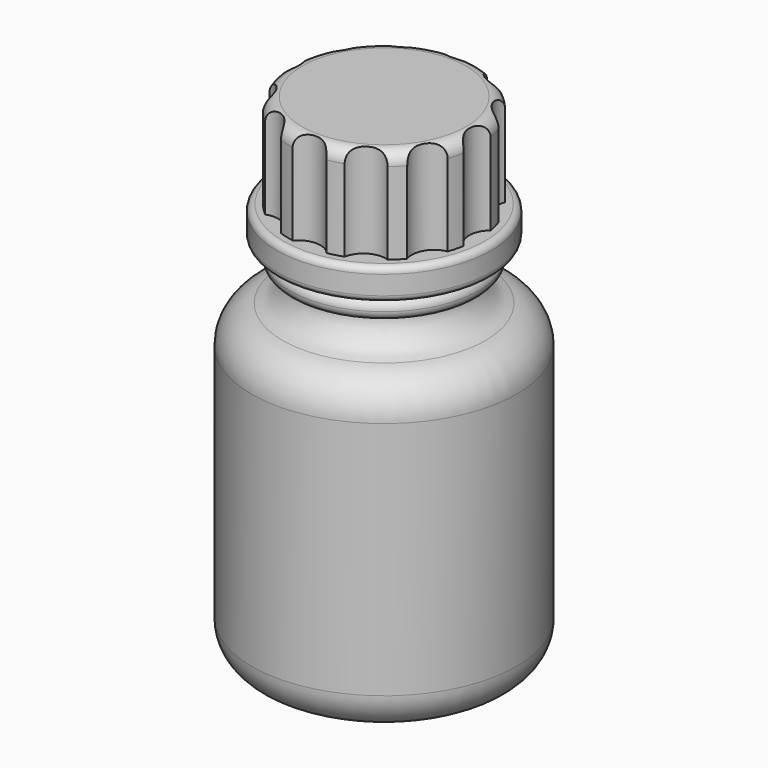
from build123d import *

# Parameters (mm, degrees)
F2_R     = 6
F3_R     = 6
F4_R     = 4.99999
F5_R     = 1.49999
F6_R     = 1
F7_R     = 2
F8_R     = 3.5
F9_DEPTH = 15


# Not quite as in the source:
# - a fillet or chamfer is up to 0.001 mm smaller than in the source, because OpenCascade refuses the exact size


with BuildPart() as f1:
    # F0 (on Front) → F1 (revolve)
    with BuildSketch(Plane.XZ):
        Polygon((-21, 0), (0, 0), (0, 78.75), (-15, 78.75), (-15, 63.75), (-17, 63.75), (-17, 58.75), (-12, 58.75), (-12, 58), (-15, 58), (-15, 55), (-12, 55), (-12, 50), (-21, 50), align=None)
    revolve(axis=Axis((0, 0, 32.9393539578), (0, 0, -1)))

    # F2
    f2_edges = [f1.edges().sort_by_distance(p)[0] for p in [
        (21, 0, 0),
    ]]
    fillet(f2_edges, radius=F2_R)

    # F3
    f3_edges = [f1.edges().sort_by_distance(p)[0] for p in [
        (21, 0, 50),
    ]]
    fillet(f3_edges, radius=F3_R)

    # F4 (radius 5 in the source; OpenCascade refuses exactly that, so slightly less here)
    f4_edges = [f1.edges().sort_by_distance(p)[0] for p in [
        (12, 0, 50),
    ]]
    fillet(f4_edges, radius=F4_R)

    # F5 (radius 1.5 in the source; OpenCascade refuses exactly that, so slightly less here)
    f5_edges = [f1.edges().sort_by_distance(p)[0] for p in [
        (15, 0, 55),
        (15, 0, 58),
    ]]
    fillet(f5_edges, radius=F5_R)

    # F6
    f6_edges = [f1.edges().sort_by_distance(p)[0] for p in [
        (17, 0, 58.75),
        (17, 0, 63.75),
    ]]
    fillet(f6_edges, radius=F6_R)

    # F7
    f7_edges = [f1.edges().sort_by_distance(p)[0] for p in [
        (15, 0, 78.75),
    ]]
    fillet(f7_edges, radius=F7_R)

    # F8 (on face) → F9 (cut)
    with BuildSketch(Plane.XY.offset(78.75)):
        with Locations((0, 17)):
            Circle(F8_R)
        with Locations((-8.5, 14.7224318643)):
            Circle(F8_R)
        with Locations((-14.7224318643, 8.5)):
            Circle(F8_R)
        with Locations((-17, 0)):
            Circle(F8_R)
        with Locations((-14.7224318643, -8.5)):
            Circle(F8_R)
        with Locations((-8.5, -14.7224318643)):
            Circle(F8_R)
        with Locations((0, -17)):
            Circle(F8_R)
        with Locations((8.5, -14.7224318643)):
            Circle(F8_R)
        with Locations((14.7224318643, -8.5)):
            Circle(F8_R)
        with Locations((17, 0)):
            Circle(F8_R)
        with Locations((14.7224318643, 8.5)):
            Circle(F8_R)
        with Locations((8.5, 14.7224318643)):
            Circle(F8_R)
    extrude(amount=-F9_DEPTH, mode=Mode.SUBTRACT)


solid = f1.part
